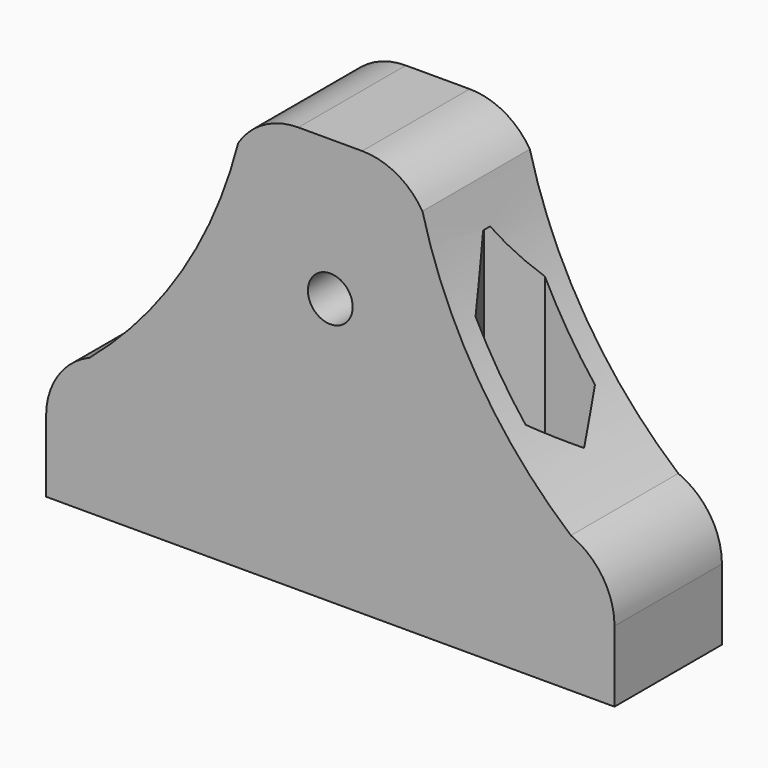
from build123d import *

# Parameters (mm, degrees)
F0_W      = 20
F0_H      = 5
F1_DEPTH  = 3
F0_H_2    = 3
F0_H_3    = 2
F2_DEPTH  = 15
F3_R      = 2
F4_DEPTH  = 2
F5_DEPTH  = 25.4
F6_R      = 2
F7_DEPTH  = 6
F8_DEPTH  = 6
F9_R      = 2
F10_DEPTH = 25.4
F11_START = 9
F11_DEPTH = 21


with BuildPart() as f1:
    # F0 (on Top) → F1 (new body)
    with BuildSketch(Plane.XY):
        with Locations((-6.108090542, -1.053064514)):
            Rectangle(F0_W, F0_H)
    extrude(amount=F1_DEPTH)

    # F0 (on Top) → F2 (join)
    with BuildSketch(Plane.XY):
        with Locations((-6.108090542, 2.946935486)):
            Rectangle(F0_W, F0_H_2)
        with Locations((-6.108090542, -4.553064514)):
            Rectangle(F0_W, F0_H_3)
    extrude(amount=F2_DEPTH)

    # F3 (on face) → F4 (cut)
    with BuildSketch(Plane(origin=(0, 4.446935486, 0), x_dir=(-1, 0, 0), z_dir=(0, 1, 0))):
        Polygon((10.5825551282, 8.9868011065), (8.3453228351, 13), (3.8708582489, 13), (1.6336259557, 8.9868011065), (3.8708582489, 5.25), (8.3453228351, 5.25), align=None)
        with Locations((6.108090542, 9.125)):
            Circle(F3_R, mode=Mode.SUBTRACT)
    extrude(amount=-F4_DEPTH, mode=Mode.SUBTRACT)

    # F5 (cut): a face of the model
    f5_faces = [f1.faces().sort_by_distance(p)[0] for p in [
        (-6.108090542, 4.446935486, 9.125),
    ]]
    extrude(f5_faces, amount=-F5_DEPTH, mode=Mode.SUBTRACT)


with BuildPart() as f7:
    # F6 (on Front) → F7 (new body)
    with BuildSketch(Plane.XZ):
        with BuildLine():
            Line((-25.4, 6.35), (-25.4, 0))
            Line((-25.4, 0), (25.4, 0))
            Line((25.4, 0), (25.4, 6.3500013265))
            ThreePointArc((25.4, 6.3500013265), (24.3368879233, 9.8672894988), (21.5035224923, 12.2068543535))
            ThreePointArc((21.5035224923, 12.2068543535), (13.2254338027, 21.7784198761), (8.233914751, 33.4071066662))
            ThreePointArc((8.233914751, 33.4071066662), (5.9277949415, 35.5930574418), (2.8513464312, 36.3880630597))
            Line((2.8513464312, 36.3880630597), (-2.8513454918, 36.3880633483))
            ThreePointArc((-2.8513454918, 36.3880633483), (-5.9277945127, 35.5930578036), (-8.233914635, 33.4071066662))
            ThreePointArc((-8.233914635, 33.4071066662), (-13.2254333146, 21.7784197643), (-21.5035211719, 12.2068535801))
            ThreePointArc((-21.5035211719, 12.2068535801), (-24.3368875268, 9.8672887683), (-25.4, 6.35))
        make_face()
        Polygon((0, 28.3061052624), (3.875, 26.0688729693), (3.8059005532, 21.4747246305), (0, 19.3571760899), (-3.875, 21.594408383), (-3.9440994468, 25.9491892167), align=None, mode=Mode.SUBTRACT)
        Polygon((3.8059005532, 21.4747246305), (3.875, 26.0688729693), (0, 28.3061052624), (-3.9440994468, 25.9491892167), (-3.875, 21.594408383), (0, 19.3571760899), align=None)
        with Locations((0, 23.8316406762)):
            Circle(F6_R, mode=Mode.SUBTRACT)
    extrude(amount=F7_DEPTH)

    # F6 (on Front) → F8 (join)
    with BuildSketch(Plane.XZ):
        with BuildLine():
            Line((-25.4, 6.35), (-25.4, 0))
            Line((-25.4, 0), (25.4, 0))
            Line((25.4, 0), (25.4, 6.3500013265))
            ThreePointArc((25.4, 6.3500013265), (24.3368879233, 9.8672894988), (21.5035224923, 12.2068543535))
            ThreePointArc((21.5035224923, 12.2068543535), (13.2254338027, 21.7784198761), (8.233914751, 33.4071066662))
            ThreePointArc((8.233914751, 33.4071066662), (5.9277949415, 35.5930574418), (2.8513464312, 36.3880630597))
            Line((2.8513464312, 36.3880630597), (-2.8513454918, 36.3880633483))
            ThreePointArc((-2.8513454918, 36.3880633483), (-5.9277945127, 35.5930578036), (-8.233914635, 33.4071066662))
            ThreePointArc((-8.233914635, 33.4071066662), (-13.2254333146, 21.7784197643), (-21.5035211719, 12.2068535801))
            ThreePointArc((-21.5035211719, 12.2068535801), (-24.3368875268, 9.8672887683), (-25.4, 6.35))
        make_face()
        Polygon((0, 28.3061052624), (3.875, 26.0688729693), (3.8059005532, 21.4747246305), (0, 19.3571760899), (-3.875, 21.594408383), (-3.9440994468, 25.9491892167), align=None, mode=Mode.SUBTRACT)
    extrude(amount=-F8_DEPTH)

    # F9 (on Top) → F10 (cut)
    with BuildSketch(Plane.XY):
        with Locations((-13.5221913382, 0)):
            Circle(F9_R)
        with Locations((13.5180821443, 0)):
            Circle(F9_R)
    extrude(amount=F10_DEPTH, mode=Mode.SUBTRACT)

    # F9 (on Top) → F11 (cut)
    with BuildSketch(Plane.XY.offset(F11_START)):
        Polygon((-9.047726752, -0.1381988935), (-11.2849590451, 3.875), (-15.7594236313, 3.875), (-17.9966559245, -0.1381988935), (-15.7594236313, -3.875), (-11.2849590451, -3.875), align=None)
        with Locations((-13.5221913382, 0)):
            Circle(F9_R, mode=Mode.SUBTRACT)
        Polygon((17.9925467305, -0.1381988935), (15.7553144374, 3.875), (11.2808498512, 3.875), (9.0436175581, -0.1381988935), (11.2808498512, -3.875), (15.7553144374, -3.875), align=None)
        with Locations((13.5180821443, 0)):
            Circle(F9_R, mode=Mode.SUBTRACT)
    extrude(amount=F11_DEPTH, mode=Mode.SUBTRACT)


solid = Compound([f1.part, f7.part])
